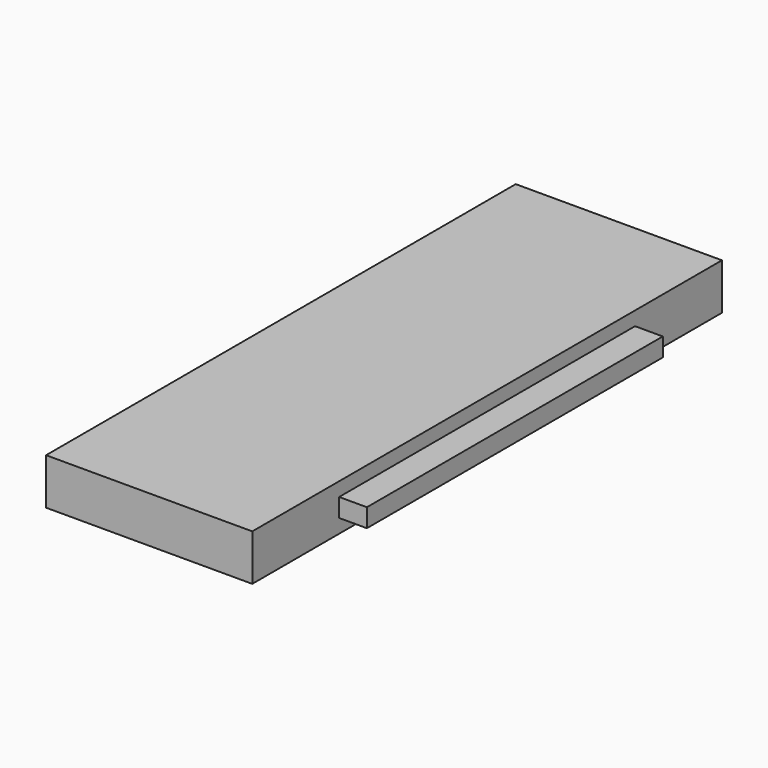
from build123d import *

# Parameters (mm, degrees)
F0_W     = 63.49
F0_H     = 5
F1_DEPTH = 22.3
F2_W     = 40
F2_H     = 2
F3_DEPTH = 3


# Not quite as in the source:
# - a feature of the source that left no trace in its solid (it failed there, or was rolled back) is left out


with BuildPart() as f1:
    # F0 (on Right) → F1 (new body)
    with BuildSketch(Plane.YZ):
        with Locations((0, 2.5)):
            Rectangle(F0_W, F0_H)
    extrude(amount=-F1_DEPTH)

    # F2 (on face) → F3 (join)
    with BuildSketch(Plane.YZ):
        with Locations((0, 2.5)):
            Rectangle(F2_W, F2_H)
    extrude(amount=F3_DEPTH)


solid = f1.part
